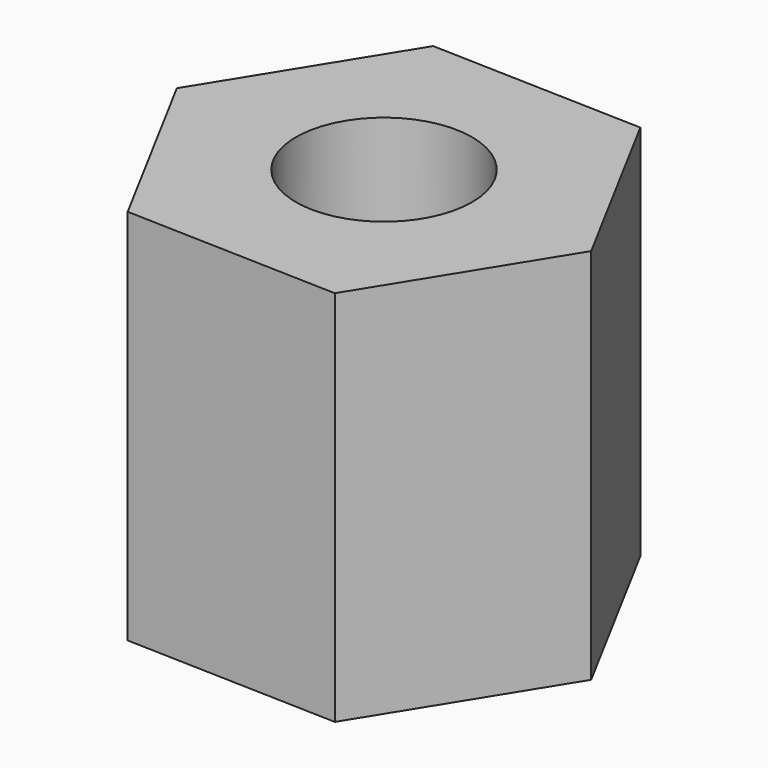
from build123d import *

# Parameters (mm, degrees)
F0_R         = 3.5
F0_R_2       = 2.8
F1_DEPTH     = 12
F3_DEPTH     = 1.7
F5_DEPTH     = 0.7
F6_T4_DEPTH  = 6.526963201
F6_S5_R      = 2.8
F6_T6_DEPTH  = 5
F6_T10_DEPTH = 6.526963201
F6_S11_R     = 2.8
F6_T12_DEPTH = 5
F6_T16_DEPTH = 6.526963201
F6_S17_R     = 2.8
F6_T18_DEPTH = 5
F6_T22_DEPTH = 6.526963201
F6_S23_R     = 2.8
F6_T24_DEPTH = 5
F7_T2_ANGLE  = 236.1398810925
F7_T4_ANGLE  = 236.1398810925


# Not quite as in the source:
# - a fillet or chamfer that OpenCascade refuses, or shapes differently, is made with other operations: its cross-section is extruded or revolved along the edge and cut away or added
# - a pattern or mirror of a feature is missing from the dataset's text; its kind, count and spacing are read off the source's solid


with BuildPart() as f1:
    # F0 (on Top) → F1 (new body)
    with BuildSketch(Plane.XY):
        Polygon((3.1971086236, -5.9505038819), (6.7518418389, -0.2064746542), (3.5547332152, 5.7440292277), (-3.1971086236, 5.9505038819), (-6.7518418389, 0.2064746542), (-3.5547332152, -5.7440292277), align=None)
        Circle(F0_R, mode=Mode.SUBTRACT)
        Circle(F0_R)
        Circle(F0_R_2, mode=Mode.SUBTRACT)
    extrude(amount=F1_DEPTH)

    # F2 (on face) → F3 (cut)
    with BuildSketch(Plane(origin=(0, 0, 0), x_dir=(1, 0, 0), z_dir=(0, 0, -1))):
        with BuildLine():
            Line((-5.3518418389, -1.1), (-2.5748786379, -1.1))
            ThreePointArc((-2.5748786379, -1.1), (-2.8, 0), (-2.5748786379, 1.1))
            Line((-2.5748786379, 1.1), (-5.3518418389, 1.1))
            Line((-5.3518418389, 1.1), (-5.3518418389, -1.1))
        make_face()
        with BuildLine():
            Line((2.5748786379, -1.1), (5.3518418389, -1.1))
            Line((5.3518418389, -1.1), (5.3518418389, 1.1))
            Line((5.3518418389, 1.1), (2.5748786379, 1.1))
            ThreePointArc((2.5748786379, 1.1), (2.7431423756, 0.5613999527), (2.8, 0))
            ThreePointArc((2.8, 0), (2.7431423756, -0.5613999527), (2.5748786379, -1.1))
        make_face()
    extrude(amount=-F3_DEPTH, mode=Mode.SUBTRACT)

    # F4 (on face) → F5 (join)
    with BuildSketch(Plane(origin=(0, 0, 0), x_dir=(1, 0, 0), z_dir=(0, 0, -1))):
        with BuildLine():
            ThreePointArc((-3.6402666737, -1.1), (0, -3.8028333457), (3.6402666737, -1.1))
            Line((3.6402666737, -1.1), (2.5748786379, -1.1))
            ThreePointArc((2.5748786379, -1.1), (0, -2.8), (-2.5748786379, -1.1))
            Line((-2.5748786379, -1.1), (-3.6402666737, -1.1))
        make_face()
    f5 = extrude(amount=F5_DEPTH)

    # F5_copies: F5 across plane
    add(f5.mirror(Plane(origin=(0, 0, 0), x_dir=(0, 0, -1), z_dir=(0, -1, 0))))

    # F6: fillet of radius 1.5 on 4 edges, made by hand


with BuildPart() as f6_tool2:
    # F6_s3 → F6_t4 (new body)
    with BuildSketch(Plane.YZ.offset(-1.1751213621)):
        with BuildLine():
            ThreePointArc((1.1, 0.2), (0.6606601718, 1.2606601718), (-0.4, 1.7))
            Line((-0.4, 1.7), (1.1, 1.7))
            Line((1.1, 1.7), (1.1, 0.2))
        make_face()
    extrude(amount=F6_T4_DEPTH)

    # F6_s5 → F6_t6 (cut, symmetric)
    with BuildSketch(Plane.XY.offset(1)):
        Circle(F6_S5_R)
    extrude(amount=F6_T6_DEPTH, both=True, mode=Mode.SUBTRACT)


with BuildPart() as f1_1:
    add(f1.part)

    # F6_t1: union F6_tool2
    add(f6_tool2.part)


with BuildPart() as f6_tool8:
    # F6_s9 → F6_t10 (new body)
    with BuildSketch(Plane.YZ.offset(-5.3518418389)):
        with BuildLine():
            ThreePointArc((1.1, 0.2), (0.6606601718, 1.2606601718), (-0.4, 1.7))
            Line((-0.4, 1.7), (1.1, 1.7))
            Line((1.1, 1.7), (1.1, 0.2))
        make_face()
    extrude(amount=F6_T10_DEPTH)

    # F6_s11 → F6_t12 (cut, symmetric)
    with BuildSketch(Plane.XY.offset(1)):
        Circle(F6_S11_R)
    extrude(amount=F6_T12_DEPTH, both=True, mode=Mode.SUBTRACT)


with BuildPart() as f1_2:
    add(f1_1.part)

    # F6_t7: union F6_tool8
    add(f6_tool8.part)


with BuildPart() as f6_tool14:
    # F6_s15 → F6_t16 (new body)
    with BuildSketch(Plane.YZ.offset(5.3518418389)):
        with BuildLine():
            ThreePointArc((-1.1, 0.2), (-0.6606601718, 1.2606601718), (0.4, 1.7))
            Line((0.4, 1.7), (-1.1, 1.7))
            Line((-1.1, 1.7), (-1.1, 0.2))
        make_face()
    extrude(amount=-F6_T16_DEPTH)

    # F6_s17 → F6_t18 (cut, symmetric)
    with BuildSketch(Plane.XY.offset(1)):
        Circle(F6_S17_R)
    extrude(amount=F6_T18_DEPTH, both=True, mode=Mode.SUBTRACT)


with BuildPart() as f1_3:
    add(f1_2.part)

    # F6_t13: union F6_tool14
    add(f6_tool14.part)


with BuildPart() as f6_tool20:
    # F6_s21 → F6_t22 (new body)
    with BuildSketch(Plane.YZ.offset(1.1751213621)):
        with BuildLine():
            ThreePointArc((-1.1, 0.2), (-0.6606601718, 1.2606601718), (0.4, 1.7))
            Line((0.4, 1.7), (-1.1, 1.7))
            Line((-1.1, 1.7), (-1.1, 0.2))
        make_face()
    extrude(amount=-F6_T22_DEPTH)

    # F6_s23 → F6_t24 (cut, symmetric)
    with BuildSketch(Plane.XY.offset(1)):
        Circle(F6_S23_R)
    extrude(amount=F6_T24_DEPTH, both=True, mode=Mode.SUBTRACT)


with BuildPart() as f1_4:
    add(f1_3.part)

    # F6_t19: union F6_tool20
    add(f6_tool20.part)

    # F7: fillet of radius 1 on 2 edges, made by hand

    # F7_s1 → F7_t2 (revolve, cut)
    with BuildSketch(Plane(origin=(0, 0, 0), x_dir=(0, 0, 1), z_dir=(-0.4705490205, -0.8823738546, 0))):
        with BuildLine():
            ThreePointArc((0.3, -2.8), (-0.4071067812, -3.0928932188), (-0.7, -3.8))
            Line((-0.7, -3.8), (-0.7, -2.8))
            Line((-0.7, -2.8), (0.3, -2.8))
        make_face()
    revolve(axis=Axis((0, 0, -0.7), (0, 0, 1)), revolution_arc=F7_T2_ANGLE, mode=Mode.SUBTRACT)

    # F7_s3 → F7_t4 (revolve, cut)
    with BuildSketch(Plane(origin=(0, 0, 0), x_dir=(0, 0, 1), z_dir=(-0.4705490205, 0.8823738546, 0))):
        with BuildLine():
            ThreePointArc((0.3, 2.8), (-0.4071067812, 3.0928932188), (-0.7, 3.8))
            Line((-0.7, 3.8), (-0.7, 2.8))
            Line((-0.7, 2.8), (0.3, 2.8))
        make_face()
    revolve(axis=Axis((0, 0, -0.7), (0, 0, -1)), revolution_arc=F7_T4_ANGLE, mode=Mode.SUBTRACT)


solid = f1_4.part
